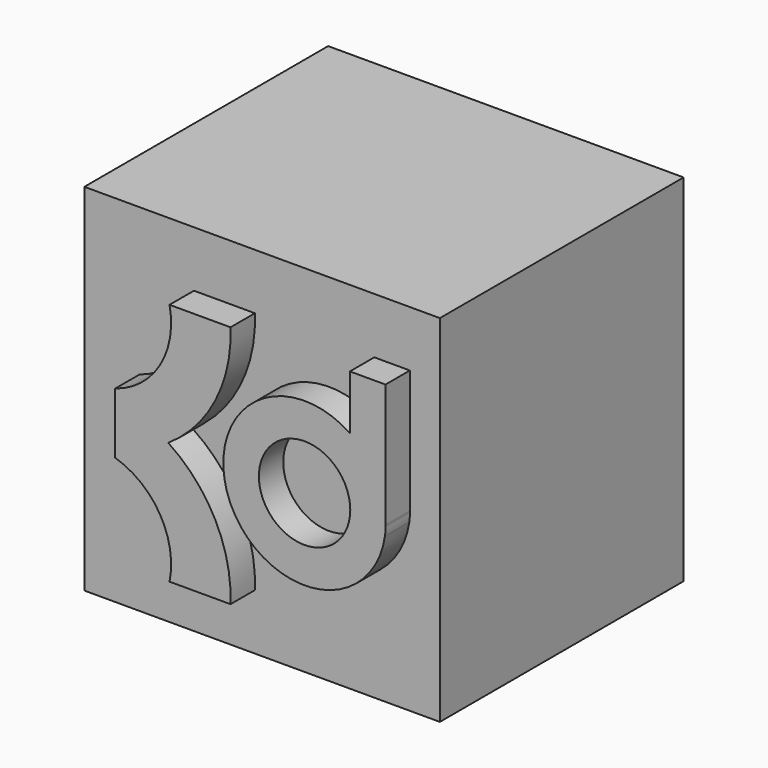
from build123d import *

# Parameters (mm, degrees)
F0_W        = 35
F0_H        = 35
F1_DEPTH    = 15
F3_R        = 4.5
F4_DEPTH    = 3
F5_T1_DEPTH = 3.9749724421
F6_R        = 5


# Not quite as in the source:
# - a fillet or chamfer that OpenCascade refuses, or shapes differently, is made with other operations: its cross-section is extruded or revolved along the edge and cut away or added


with BuildPart() as f1:
    # F0 (on Front) → F1 (new body, symmetric)
    with BuildSketch(Plane.XZ):
        Rectangle(F0_W, F0_H)
    extrude(amount=F1_DEPTH, both=True)

    # F3 (on face) → F4 (join)
    with BuildSketch(Plane.XZ.offset(15)):
        with BuildLine():
            Line((-12.0646512398, 3), (-12.0646512398, 0))
            Line((-12.0646512398, 0), (-12.0646512398, -3))
            ThreePointArc((-12.0646512398, -3), (-7.6541876394, -6.4685364284), (-6.7129943114, -12))
            Line((-6.7129943114, -12), (-0.7129943114, -12))
            ThreePointArc((-0.7129943114, -12), (-2.1988842528, -5.1949035825), (-6.8389470689, 0))
            ThreePointArc((-6.8389470689, 0), (-2.1988842528, 5.1949035825), (-0.7129943114, 12))
            Line((-0.7129943114, 12), (-6.7129943114, 12))
            ThreePointArc((-6.7129943114, 12), (-7.6541876394, 6.4685364284), (-12.0646512398, 3))
        make_face()
        with BuildLine():
            Line((11.0439136906, 12), (11.0439136906, 6.6378525317))
            ThreePointArc((11.0439136906, 6.6378525317), (-0.6094940203, -3.5115698933), (14.5591460332, -0.5577510491))
            Line((14.5591460332, -0.5577510491), (14.5439136906, -0.5577510491))
            Line((14.5439136906, -0.5577510491), (14.5439136906, 12))
            Line((14.5439136906, 12), (11.0439136906, 12))
        make_face()
        with Locations((6.578612607, 0)):
            Circle(F3_R, mode=Mode.SUBTRACT)
    extrude(amount=F4_DEPTH)

    # F5: fillet of radius 5 on 1 edges, made by hand

    # F5_s2 → F5_t1 (join)
    with BuildSketch(Plane.XZ.offset(14.0250275579)):
        with BuildLine():
            ThreePointArc((14.5591460332, -0.5577510491), (14.5477232275, -0.3629052417), (14.5439136906, -0.1677620723))
            Line((14.5439136906, -0.1677620723), (14.5439136906, -0.5577510491))
            Line((14.5439136906, -0.5577510491), (14.5591460332, -0.5577510491))
        make_face()
    extrude(amount=F5_T1_DEPTH)

    # F6
    f6_edges = [f1.edges().sort_by_distance(p)[0] for p in [
        (14.559146, -16.5, -0.557751),
    ]]
    fillet(f6_edges, radius=F6_R)


solid = f1.part
